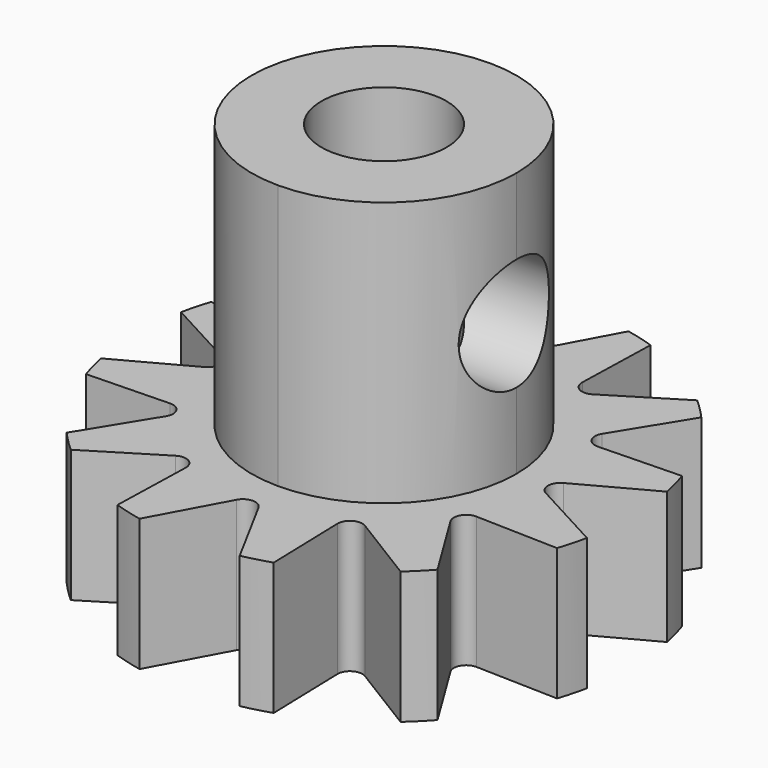
from build123d import *

# Parameters (mm, degrees)
F0_R        = 5.9508004686
F0_R_2      = 1.5
F1_DEPTH    = 3.175
F2_W        = 6.35
F2_H        = 6.35
F2_R        = 1.5
F3_DEPTH    = 6.35
F4_R        = 1.35255
F5_REACH    = 12.9523895761
F6_T1_DEPTH = 6.35
F8_DEPTH    = 3.175
F9_COUNT    = 12
F9_ANGLE    = 330


# Not quite as in the source:
# - a fillet or chamfer that OpenCascade refuses, or shapes differently, is made with other operations: its cross-section is extruded or revolved along the edge and cut away or added


with BuildPart() as f1:
    # F0 (on Top) → F1 (new body)
    with BuildSketch(Plane.XY):
        Circle(F0_R)
        Circle(F0_R_2, mode=Mode.SUBTRACT)
    extrude(amount=F1_DEPTH)

    # F2 (on face) → F3 (join)
    with BuildSketch(Plane.XY.offset(3.175)):
        Rectangle(F2_W, F2_H)
        Circle(F2_R, mode=Mode.SUBTRACT)
    extrude(amount=F3_DEPTH)

    f5_end = f1.faces().sort_by_distance((-1.5, 0, 4.7625))[0]
    # F4 (on face) → F5 (cut, up to a face of the model that its end follows)
    with BuildSketch(Plane.YZ.offset(3.175)):
        with Locations((0, 6.35)):
            Circle(F4_R)
    f5_long = extrude(amount=-F5_REACH, mode=Mode.PRIVATE)
    add(split(f5_long, bisect_by=f5_end, keep=Keep.ALL, mode=Mode.PRIVATE).solids().sort_by_distance((3.175, 0, 6.35))[0], mode=Mode.SUBTRACT)

    # F6: fillet of radius 3.175 on 4 edges, made by hand

    # F6_s2 → F6_t1 (cut)
    with BuildSketch(Plane.XY.offset(3.175)):
        with BuildLine():
            ThreePointArc((0, -3.175), (2.2450640303, -2.2450640303), (3.175, 0))
            Line((3.175, 0), (3.2385, 0))
            Line((3.2385, 0), (3.2385, -3.2385))
            Line((3.2385, -3.2385), (0, -3.2385))
            Line((0, -3.2385), (0, -3.175))
        make_face()
        with BuildLine():
            ThreePointArc((0, -3.175), (-2.2450640303, -2.2450640303), (-3.175, 0))
            Line((-3.175, 0), (-3.2385, 0))
            Line((-3.2385, 0), (-3.2385, -3.2385))
            Line((-3.2385, -3.2385), (0, -3.2385))
            Line((0, -3.2385), (0, -3.175))
        make_face()
        with BuildLine():
            ThreePointArc((3.175, 0), (2.2450640303, 2.2450640303), (0, 3.175))
            Line((0, 3.175), (0, 3.2385))
            Line((0, 3.2385), (3.2385, 3.2385))
            Line((3.2385, 3.2385), (3.2385, 0))
            Line((3.2385, 0), (3.175, 0))
        make_face()
        with BuildLine():
            ThreePointArc((0, 3.175), (-2.2450640303, 2.2450640303), (-3.175, 0))
            Line((-3.175, 0), (-3.2385, 0))
            Line((-3.2385, 0), (-3.2385, 3.2385))
            Line((-3.2385, 3.2385), (0, 3.2385))
            Line((0, 3.2385), (0, 3.175))
        make_face()
    extrude(amount=F6_T1_DEPTH, mode=Mode.SUBTRACT)

    # F7 (on face) → F8 (cut, through all)
    with BuildSketch(Plane(origin=(0, 0, 0), x_dir=(1, 0, 0), z_dir=(0, 0, -1))):
        with BuildLine():
            Line((4.0897477961, -0.2617496271), (5.8282529848, -1.2014546857))
            ThreePointArc((5.8282529848, -1.2014546857), (5.9508004686, 0), (5.8282529848, 1.2014546857))
            Line((5.8282529848, 1.2014546857), (4.0897477961, 0.2617496271))
            ThreePointArc((4.0897477961, 0.2617496271), (3.9336899209, 0), (4.0897477961, -0.2617496271))
        make_face()
    f8 = extrude(amount=-F8_DEPTH, mode=Mode.SUBTRACT)

    # F9: F8 ×12 about axis
    f9_axis = Axis((0, 0, 0), (0, 0, -1))
    for i in range(1, F9_COUNT):
        add(f8.rotate(f9_axis, i * F9_ANGLE / (F9_COUNT - 1)), mode=Mode.SUBTRACT)


solid = f1.part
